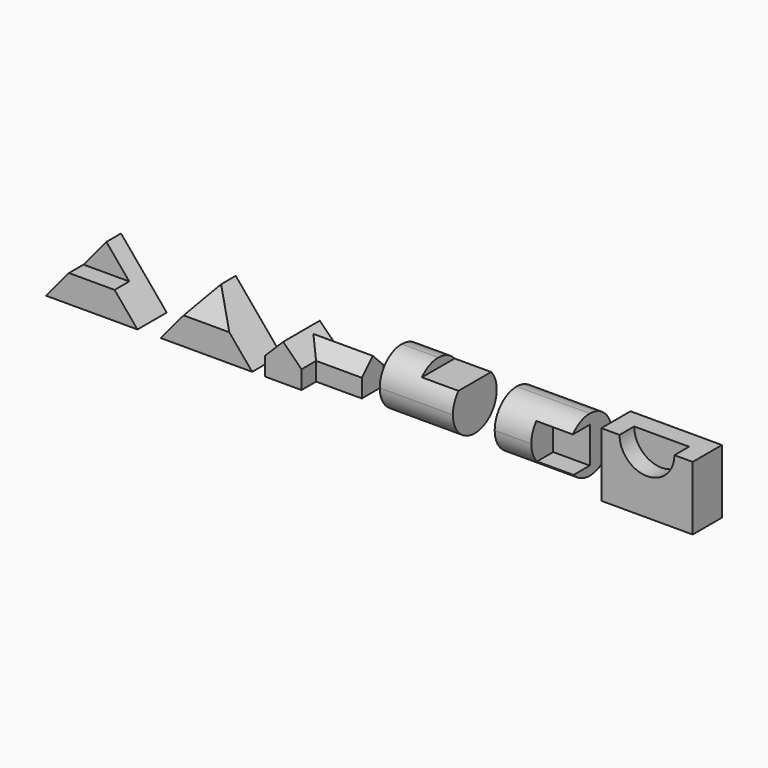
from build123d import *

# Parameters (mm, degrees)
F0_W      = 254
F0_H      = 152.4
F1_DEPTH  = 101.6
F3_DEPTH  = 171.45
F5_DEPTH  = 50.8
F7_DEPTH  = 181.102
F8_W      = 254
F8_H      = 152.4
F9_DEPTH  = 101.6
F11_DEPTH = 317.754
F13_DEPTH = 144.78
F15_DEPTH = 111.76
F16_W     = 228.6
F16_H     = 127
F17_DEPTH = 101.6
F18_W     = 127
F18_H     = 50.8
F19_DEPTH = 124.46
F20_W     = 76.2
F20_H     = 12.7
F21_DEPTH = 127
F23_DEPTH = 210.82
F25_DEPTH = 127
F27_DEPTH = 127
F29_DEPTH = 157.48
F31_DEPTH = 177.8
F32_W     = 203.2
F32_H     = 152.4
F33_DEPTH = 152.4
F34_W     = 152.4
F34_H     = 25.4
F35_DEPTH = 101.6
F36_R     = 76.2
F37_R     = 76.19999
F38_R     = 76.19999
F39_R     = 76.2
F40_W     = 203.2
F40_H     = 152.4
F41_DEPTH = 152.4
F42_W     = 101.5413056934
F42_H     = 99.8808480799
F43_DEPTH = 76.2
F44_R     = 76.2
F45_R     = 76.19999
F46_W     = 254
F46_H     = 101.6
F47_DEPTH = 177.8
F49_DEPTH = 50.8


# Not quite as in the source:
# - a fillet or chamfer is up to 0.001 mm smaller than in the source, because OpenCascade refuses the exact size


with BuildPart() as f1:
    # F0 (on Front) → F1 (new body)
    with BuildSketch(Plane.XZ):
        with Locations((230.1876775126, 76.2)):
            Rectangle(F0_W, F0_H)
    extrude(amount=-F1_DEPTH)

    # F2 (on face) → F3 (cut)
    with BuildSketch(Plane.XZ):
        Polygon((103.1876775126, 152.4), (103.1876775126, 0), (166.6876775126, 76.2), (230.1876775126, 152.4), align=None)
    extrude(amount=-F3_DEPTH, mode=Mode.SUBTRACT)

    # F4 (on face) → F5 (cut)
    with BuildSketch(Plane.XZ):
        Polygon((166.6876775126, 76.2), (293.6876775126, 76.2), (230.1876775126, 152.4), align=None)
    extrude(amount=-F5_DEPTH, mode=Mode.SUBTRACT)

    # F6 (on face) → F7 (cut)
    with BuildSketch(Plane.XZ):
        Polygon((230.1876775126, 152.4), (293.6876775126, 76.2), (357.1876775126, 0), (357.1876775126, 152.4), align=None)
    extrude(amount=-F7_DEPTH, mode=Mode.SUBTRACT)


with BuildPart() as f9:
    # F8 (on Front) → F9 (new body)
    with BuildSketch(Plane.XZ):
        with Locations((548.9165070272, 76.2)):
            Rectangle(F8_W, F8_H)
    extrude(amount=-F9_DEPTH)

    # F10 (on face) → F11 (cut)
    with BuildSketch(Plane.YZ.offset(675.9165070272)):
        Polygon((0, 152.4), (0, 76.2), (50.8, 152.4), align=None)
    extrude(amount=-F11_DEPTH, mode=Mode.SUBTRACT)

    # F12 (on face) → F13 (cut)
    with BuildSketch(Plane(origin=(0, 101.6, 0), x_dir=(-1, 0, 0), z_dir=(0, 1, 0))):
        Polygon((-675.9165070272, 152.4), (-675.9165070272, 0), (-548.9165070272, 152.4), align=None)
    extrude(amount=-F13_DEPTH, mode=Mode.SUBTRACT)

    # F14 (on face) → F15 (cut)
    with BuildSketch(Plane(origin=(0, 101.6, 0), x_dir=(-1, 0, 0), z_dir=(0, 1, 0))):
        Polygon((-421.9165070272, 152.4), (-548.9165070272, 152.4), (-421.9165070272, 0), align=None)
    extrude(amount=-F15_DEPTH, mode=Mode.SUBTRACT)


with BuildPart() as f17:
    # F16 (on Top) → F17 (new body)
    with BuildSketch(Plane.XY):
        with Locations((825.6324577618, 63.5)):
            Rectangle(F16_W, F16_H)
    extrude(amount=F17_DEPTH)

    # F18 (on face) → F19 (cut)
    with BuildSketch(Plane.XY.offset(101.6)):
        with Locations((876.4324577618, 25.4)):
            Rectangle(F18_W, F18_H)
    extrude(amount=-F19_DEPTH, mode=Mode.SUBTRACT)

    # F20 (on face) → F21 (cut)
    with BuildSketch(Plane.YZ.offset(939.9324577618)):
        with Locations((88.9, 95.25)):
            Rectangle(F20_W, F20_H)
    extrude(amount=-F21_DEPTH, mode=Mode.SUBTRACT)

    # F22 (on face) → F23 (cut)
    with BuildSketch(Plane.XZ):
        Polygon((711.3324577618, 50.8), (762.1324577618, 101.6), (711.3324577618, 101.6), align=None)
    extrude(amount=-F23_DEPTH, mode=Mode.SUBTRACT)

    # F24 (on face) → F25 (cut)
    with BuildSketch(Plane.YZ.offset(939.9324577618)):
        Polygon((88.9, 88.9), (127, 50.8), (127, 88.9), align=None)
    extrude(amount=-F25_DEPTH, mode=Mode.SUBTRACT)

    # F26 (on face) → F27 (cut)
    with BuildSketch(Plane.YZ.offset(939.9324577618)):
        Polygon((50.8, 88.9), (50.8, 50.8), (88.9, 88.9), align=None)
    extrude(amount=-F27_DEPTH, mode=Mode.SUBTRACT)

    # F28 (on face) → F29 (cut)
    with BuildSketch(Plane.XZ):
        Polygon((762.1324577618, 101.6), (812.9324577618, 50.8), (812.9324577618, 101.6), align=None)
    extrude(amount=-F29_DEPTH, mode=Mode.SUBTRACT)

    # F30 (on face) → F31 (join)
    with BuildSketch(Plane.YZ.offset(939.9324577618)):
        Polygon((88.9, 88.9), (50.8, 50.8), (127, 50.8), align=None)
    extrude(amount=-F31_DEPTH)


with BuildPart() as f33:
    # F32 (on Top) → F33 (new body)
    with BuildSketch(Plane.XY):
        with Locations((1132.0576660588, 76.2)):
            Rectangle(F32_W, F32_H)
    extrude(amount=F33_DEPTH)

    # F34 (on face) → F35 (cut)
    with BuildSketch(Plane.YZ.offset(1233.6576660588)):
        with Locations((76.2, 139.7)):
            Rectangle(F34_W, F34_H)
    extrude(amount=-F35_DEPTH, mode=Mode.SUBTRACT)

    # F36
    f36_edges = [f33.edges().sort_by_distance(p)[0] for p in [
        (1081.257666, 152.4, 152.4),
    ]]
    fillet(f36_edges, radius=F36_R)

    # F37 (radius 76.2 in the source; OpenCascade refuses exactly that, so slightly less here)
    f37_edges = [f33.edges().sort_by_distance(p)[0] for p in [
        (1081.257666, 0, 152.4),
    ]]
    fillet(f37_edges, radius=F37_R)

    # F38 (radius 76.2 in the source; OpenCascade refuses exactly that, so slightly less here)
    f38_edges = [f33.edges().sort_by_distance(p)[0] for p in [
        (1132.057666, 152.4, 0),
    ]]
    fillet(f38_edges, radius=F38_R)

    # F39
    f39_edges = [f33.edges().sort_by_distance(p)[0] for p in [
        (1132.057666, 0, 0),
    ]]
    fillet(f39_edges, radius=F39_R)


with BuildPart() as f41:
    # F40 (on Top) → F41 (new body)
    with BuildSketch(Plane.XY):
        with Locations((1451.4601989353, 76.2)):
            Rectangle(F40_W, F40_H)
    extrude(amount=F41_DEPTH)

    # F42 (on face) → F43 (cut)
    with BuildSketch(Plane.XZ):
        with Locations((1502.2895460886, 74.9775152653)):
            Rectangle(F42_W, F42_H)
    extrude(amount=-F43_DEPTH, mode=Mode.SUBTRACT)

    # F44
    f44_edges = [f41.edges().sort_by_distance(p)[0] for p in [
        (1451.460199, 0, 152.4),
    ]]
    fillet(f44_edges, radius=F44_R)

    # F45 (radius 76.2 in the source; OpenCascade refuses exactly that, so slightly less here)
    f45_edges = [f41.edges().sort_by_distance(p)[0] for p in [
        (1451.460199, 0, 0),
        (1451.460199, 152.4, 152.4),
        (1451.460199, 152.4, 0),
    ]]
    fillet(f45_edges, radius=F45_R)


with BuildPart() as f47:
    # F46 (on Top) → F47 (new body)
    with BuildSketch(Plane.XY):
        with Locations((1773.0333075482, 50.8)):
            Rectangle(F46_W, F46_H)
    extrude(amount=F47_DEPTH)

    # F48 (on face) → F49 (cut)
    with BuildSketch(Plane.XZ):
        with BuildLine():
            ThreePointArc((1696.8333075482, 177.8), (1773.0333075482, 101.6), (1849.2333075482, 177.8))
            Line((1849.2333075482, 177.8), (1696.8333075482, 177.8))
        make_face()
    extrude(amount=-F49_DEPTH, mode=Mode.SUBTRACT)


solid = Compound([f1.part, f9.part, f17.part, f33.part, f41.part, f47.part])
